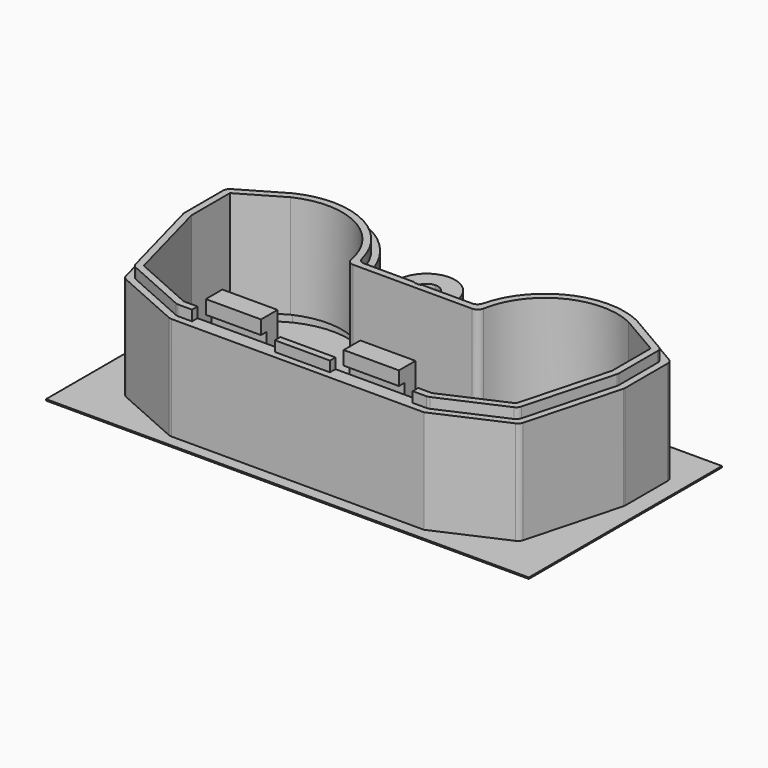
from build123d import *

# Parameters (mm, degrees)
F1_DEPTH       = 1.5
F2_DEPTH       = 15
F3_R           = 1
F5_DEPTH       = 1.5
F6_W           = 11
F6_H           = 1.5
F7_DEPTH       = 1
F8_W           = 10
F8_H           = 3
F9_DEPTH       = 1
F10_W          = 8
F10_H          = 1
F10_H_2        = 2
F11_DEPTH      = 5
F11_DEPTH_BACK = 2
F12_W          = 12
F12_H          = 1.5
F13_DEPTH      = 1
F14_W          = 70
F14_H          = 35
F15_DEPTH      = 0.2
F14_W_2        = 47
F14_H_2        = 15


with BuildPart() as f1:
    # F0 (on Top) → F1 (new body)
    with BuildSketch(Plane.XY):
        with BuildLine():
            ThreePointArc((0, 19.85), (-0.351781182, 19.8879361055), (-0.6873863542, 20))
            Line((-0.6873863542, 20), (-8.6247335107, 20))
            ThreePointArc((-8.6247335107, 20), (-14.7071371013, 28.2669276783), (-24.9698908295, 28.3836006819))
            Line((-24.9698908295, 28.3836006819), (-31.5, 24.5743703325))
            Line((-31.5, 24.5743703325), (-31.5, 16.8677394235))
            Line((-31.5, 16.8677394235), (-27.8417010277, 3.2797718121))
            Line((-27.8417010277, 3.2797718121), (-18.2122144504, -1))
            Line((-18.2122144504, -1), (0, -1))
            Line((0, -1), (18.2122144504, -1))
            Line((18.2122144504, -1), (27.8417010277, 3.2797718121))
            Line((27.8417010277, 3.2797718121), (31.5, 16.8677394235))
            Line((31.5, 16.8677394235), (31.5, 24.5743703325))
            Line((31.5, 24.5743703325), (24.9698908295, 28.3836006819))
            ThreePointArc((24.9698908295, 28.3836006819), (14.7071371013, 28.2669276783), (8.6247335107, 20))
            Line((8.6247335107, 20), (0.6873863542, 20))
            ThreePointArc((0.6873863542, 20), (0.351781182, 19.8879361055), (0, 19.85))
        make_face()
        with BuildLine():
            Line((0, 0), (-18, 0))
            Line((-18, 0), (-27, 4))
            Line((-27, 4), (-30.5, 17))
            Line((-30.5, 17), (-30.5, 24))
            Line((-30.5, 24), (-24.5, 27.5))
            ThreePointArc((-24.5, 27.5), (-14.7788745368, 27.1696331703), (-9.5, 19))
            Line((-9.5, 19), (0, 19))
            Line((0, 19), (9.5, 19))
            ThreePointArc((9.5, 19), (14.7788745368, 27.1696331703), (24.5, 27.5))
            Line((24.5, 27.5), (30.5, 24))
            Line((30.5, 24), (30.5, 17))
            Line((30.5, 17), (27, 4))
            Line((27, 4), (18, 0))
            Line((18, 0), (0, 0))
        make_face(mode=Mode.SUBTRACT)
    extrude(amount=F1_DEPTH)

    # F0 (on Top) + F1_face (on face) → F2 (join)
    with BuildSketch(Plane.XY):
        with BuildLine():
            Line((-28.6834020554, 2.5595436242), (-18.4244289009, -2))
            Line((-18.4244289009, -2), (0, -2))
            Line((0, -2), (18.4244289009, -2))
            Line((18.4244289009, -2), (28.6834020554, 2.5595436242))
            Line((28.6834020554, 2.5595436242), (32.5, 16.735478847))
            Line((32.5, 16.735478847), (32.5, 25.1487406649))
            Line((32.5, 25.1487406649), (25.4412317406, 29.2663554829))
            ThreePointArc((25.4412317406, 29.2663554829), (14.6485898576, 29.3519368457), (7.8123925294, 21))
            Line((7.8123925294, 21), (4.119769411, 21))
            ThreePointArc((4.119769411, 21), (3.1062437123, 24.2520446944), (0, 25.65))
            ThreePointArc((0, 25.65), (-3.1062437123, 24.2520446944), (-4.119769411, 21))
            Line((-4.119769411, 21), (-7.8123925294, 21))
            ThreePointArc((-7.8123925294, 21), (-14.6485898576, 29.3519368457), (-25.4412317406, 29.2663554829))
            Line((-25.4412317406, 29.2663554829), (-32.5, 25.1487406649))
            Line((-32.5, 25.1487406649), (-32.5, 16.735478847))
            Line((-32.5, 16.735478847), (-28.6834020554, 2.5595436242))
        make_face()
        with BuildLine():
            ThreePointArc((-0.6873863542, 20), (-1.6120638945, 21.851781182), (0, 23.15))
            ThreePointArc((0, 23.15), (1.6120638945, 21.851781182), (0.6873863542, 20))
            Line((0.6873863542, 20), (8.6247335107, 20))
            ThreePointArc((8.6247335107, 20), (14.7071371013, 28.2669276783), (24.9698908295, 28.3836006819))
            Line((24.9698908295, 28.3836006819), (31.5, 24.5743703325))
            Line((31.5, 24.5743703325), (31.5, 16.8677394235))
            Line((31.5, 16.8677394235), (27.8417010277, 3.2797718121))
            Line((27.8417010277, 3.2797718121), (18.2122144504, -1))
            Line((18.2122144504, -1), (0, -1))
            Line((0, -1), (-18.2122144504, -1))
            Line((-18.2122144504, -1), (-27.8417010277, 3.2797718121))
            Line((-27.8417010277, 3.2797718121), (-31.5, 16.8677394235))
            Line((-31.5, 16.8677394235), (-31.5, 24.5743703325))
            Line((-31.5, 24.5743703325), (-24.9698908295, 28.3836006819))
            ThreePointArc((-24.9698908295, 28.3836006819), (-14.7071371013, 28.2669276783), (-8.6247335107, 20))
            Line((-8.6247335107, 20), (-0.6873863542, 20))
        make_face(mode=Mode.SUBTRACT)
    with BuildSketch(Plane(origin=(0, 14.0196943872, 0), x_dir=(1, 0, 0), z_dir=(0, 0, -1))):
        with BuildLine():
            Line((31.5, -10.5546759452), (31.5, -2.8480450363))
            Line((31.5, -2.8480450363), (27.8417010277, 10.7399225751))
            Line((27.8417010277, 10.7399225751), (18.2122144504, 15.0196943872))
            Line((18.2122144504, 15.0196943872), (-18.2122144504, 15.0196943872))
            Line((-18.2122144504, 15.0196943872), (-27.8417010277, 10.7399225751))
            Line((-27.8417010277, 10.7399225751), (-31.5, -2.8480450363))
            Line((-31.5, -2.8480450363), (-31.5, -10.5546759452))
            Line((-31.5, -10.5546759452), (-24.9698908295, -14.3639062947))
            ThreePointArc((-24.9698908295, -14.3639062947), (-14.7071371013, -14.2472332911), (-8.6247335107, -5.9803056128))
            Line((-8.6247335107, -5.9803056128), (-0.6873863542, -5.9803056128))
            ThreePointArc((-0.6873863542, -5.9803056128), (0, -5.8303056128), (0.6873863542, -5.9803056128))
            Line((0.6873863542, -5.9803056128), (8.6247335107, -5.9803056128))
            ThreePointArc((8.6247335107, -5.9803056128), (14.7071371013, -14.2472332911), (24.9698908295, -14.3639062947))
            Line((24.9698908295, -14.3639062947), (31.5, -10.5546759452))
        make_face()
        with BuildLine():
            Line((-27, 10.0196943872), (-18, 14.0196943872))
            Line((-18, 14.0196943872), (18, 14.0196943872))
            Line((18, 14.0196943872), (27, 10.0196943872))
            Line((27, 10.0196943872), (30.5, -2.9803056128))
            Line((30.5, -2.9803056128), (30.5, -9.9803056128))
            Line((30.5, -9.9803056128), (24.5, -13.4803056128))
            ThreePointArc((24.5, -13.4803056128), (14.7788745368, -13.1499387831), (9.5, -4.9803056128))
            Line((9.5, -4.9803056128), (-9.5, -4.9803056128))
            ThreePointArc((-9.5, -4.9803056128), (-14.7788745368, -13.1499387831), (-24.5, -13.4803056128))
            Line((-24.5, -13.4803056128), (-30.5, -9.9803056128))
            Line((-30.5, -9.9803056128), (-30.5, -2.9803056128))
            Line((-30.5, -2.9803056128), (-27, 10.0196943872))
        make_face(mode=Mode.SUBTRACT)
    extrude(amount=-F2_DEPTH, dir=(0, 0, 1))

    # F3
    f3_edges = [f1.edges().sort_by_distance(p)[0] for p in [
        (7.812393, 21, -7.5),
        (-7.812393, 21, -7.5),
        (-4.119769, 21, -7.5),
        (4.119769, 21, -7.5),
        (32.5, 25.148741, -7.5),
        (32.5, 16.735479, -7.5),
        (28.683402, 2.559544, -7.5),
        (-18.424429, -2, -7.5),
        (-28.683402, 2.559544, -7.5),
        (-32.5, 16.735479, -7.5),
        (-32.5, 25.148741, -7.5),
        (31.5, 24.57437, 0.75),
        (31.5, 16.867739, 0.75),
        (27.841701, 3.279772, 0.75),
        (18.212214, -1, 0.75),
        (-18.212214, -1, 0.75),
        (-27.841701, 3.279772, 0.75),
        (-31.5, 16.867739, 0.75),
        (-31.5, 24.57437, 0.75),
        (-8.624734, 20, 0.75),
        (8.624734, 20, 0.75),
        (9.5, 19, 0.75),
        (9.5, 19, -7.5),
        (-9.5, 19, 0.75),
        (-9.5, 19, -7.5),
    ]]
    fillet(f3_edges, radius=F3_R)

    # F4 (on face) → F5 (cut)
    with BuildSketch(Plane(origin=(0, 0, -15), x_dir=(1, 0, 0), z_dir=(0, 0, -1))):
        with BuildLine():
            Line((27.8417010277, -3.2797718121), (18.2122144504, 1))
            Line((18.2122144504, 1), (-18.2122144504, 1))
            Line((-18.2122144504, 1), (-27.8417010277, -3.2797718121))
            Line((-27.8417010277, -3.2797718121), (-31.5, -16.8677394235))
            Line((-31.5, -16.8677394235), (-31.5, -24.5743703325))
            Line((-31.5, -24.5743703325), (-24.9698908295, -28.3836006819))
            ThreePointArc((-24.9698908295, -28.3836006819), (-14.7071371013, -28.2669276783), (-8.6247335107, -20))
            Line((-8.6247335107, -20), (8.6247335107, -20))
            ThreePointArc((8.6247335107, -20), (14.7071371013, -28.2669276783), (24.9698908295, -28.3836006819))
            Line((24.9698908295, -28.3836006819), (31.5, -24.5743703325))
            Line((31.5, -24.5743703325), (31.5, -16.8677394235))
            Line((31.5, -16.8677394235), (27.8417010277, -3.2797718121))
        make_face()
    extrude(amount=-F5_DEPTH, mode=Mode.SUBTRACT)

    # F6 (on face) → F7 (join, through all)
    with BuildSketch(Plane(origin=(0, 0, 0), x_dir=(-1, 0, 0), z_dir=(0, 1, 0))):
        with Locations((10, -14.25)):
            Rectangle(F6_W, F6_H)
        with Locations((-10, -14.25)):
            Rectangle(F6_W, F6_H)
    extrude(amount=-F7_DEPTH)

    # F8 (on face) → F9 (cut)
    with BuildSketch(Plane(origin=(0, 0, 0), x_dir=(-1, 0, 0), z_dir=(0, 1, 0))):
        with Locations((-10, -12.5)):
            Rectangle(F8_W, F8_H)
        with Locations((10, -12.5)):
            Rectangle(F8_W, F8_H)
    extrude(amount=-F9_DEPTH, mode=Mode.SUBTRACT)

    # F10 (on face) → F11 (join, two sides)
    with BuildSketch(Plane.XY.offset(1.5)) as f11_sk:
        with Locations((10, -0.5)):
            Rectangle(F10_W, F10_H)
        with Locations((-10, -0.5)):
            Rectangle(F10_W, F10_H)
        with Locations((-10, 1)):
            Rectangle(F10_W, F10_H_2)
        with Locations((10, 1)):
            Rectangle(F10_W, F10_H_2)
    extrude(amount=-F11_DEPTH)
    extrude(f11_sk.sketch, amount=F11_DEPTH_BACK)

    # F12 (on face) → F13 (cut)
    with BuildSketch(Plane.XZ.offset(1)):
        with Locations((-10, 0.75)):
            Rectangle(F12_W, F12_H)
        with Locations((10, 0.75)):
            Rectangle(F12_W, F12_H)
    extrude(amount=-F13_DEPTH, mode=Mode.SUBTRACT)


with BuildPart() as f15:
    # F14 (on face) → F15 (new body)
    with BuildSketch(Plane(origin=(0, 0, -15), x_dir=(1, 0, 0), z_dir=(0, 0, -1))):
        with Locations((0, -13.7961478531)):
            Rectangle(F14_W, F14_H)
        with BuildLine():
            Line((-28.2478394938, -2.3659602635), (-18.6183529165, 1.9138115486))
            ThreePointArc((-18.6183529165, 1.9138115486), (-18.419805938, 1.9782156073), (-18.2122144504, 2))
            Line((-18.2122144504, 2), (18.4244289009, 2))
            Line((18.4244289009, 2), (28.2478394938, -2.3659602635))
            ThreePointArc((28.2478394938, -2.3659602635), (28.6015059173, -2.629620653), (28.8073167862, -3.0197983387))
            Line((28.8073167862, -3.0197983387), (32.4656157585, -16.60776595))
            ThreePointArc((32.4656157585, -16.60776595), (32.4913666725, -16.7366206958), (32.5, -16.8677394235))
            Line((32.5, -16.8677394235), (32.5, -24.5743703325))
            ThreePointArc((32.5, -24.5743703325), (32.3671421526, -25.0724310589), (32.0038710255, -25.4381492334))
            Line((32.0038710255, -25.4381492334), (25.4412317406, -29.2663554829))
            ThreePointArc((25.4412317406, -29.2663554829), (14.9825022619, -29.5025835286), (8.0069708388, -21.7062518681))
            ThreePointArc((8.0069708388, -21.7062518681), (7.6453319845, -21.1957151836), (7.0510879824, -21))
            Line((7.0510879824, -21), (5.1256706878, -21))
            ThreePointArc((5.1256706878, -21), (4.4537657015, -21.2593626466), (4.1303948261, -21.9029126214))
            ThreePointArc((4.1303948261, -21.9029126214), (0, -25.65), (-4.1303948261, -21.9029126214))
            ThreePointArc((-4.1303948261, -21.9029126214), (-4.4537657015, -21.2593626466), (-5.1256706878, -21))
            Line((-5.1256706878, -21), (-7.0510879824, -21))
            ThreePointArc((-7.0510879824, -21), (-7.6453319845, -21.1957151836), (-8.0069708388, -21.7062518681))
            ThreePointArc((-8.0069708388, -21.7062518681), (-14.9825022619, -29.5025835286), (-25.4412317406, -29.2663554829))
            Line((-25.4412317406, -29.2663554829), (-32.0038710255, -25.4381492334))
            ThreePointArc((-32.0038710255, -25.4381492334), (-32.3671421526, -25.0724310589), (-32.5, -24.5743703325))
            Line((-32.5, -24.5743703325), (-32.5, -16.8677394235))
            ThreePointArc((-32.5, -16.8677394235), (-32.4913666725, -16.7366206958), (-32.4656157585, -16.60776595))
            Line((-32.4656157585, -16.60776595), (-28.8073167862, -3.0197983387))
            ThreePointArc((-28.8073167862, -3.0197983387), (-28.6015059173, -2.629620653), (-28.2478394938, -2.3659602635))
        make_face(mode=Mode.SUBTRACT)
    extrude(amount=F15_DEPTH)


with BuildPart() as f15b:
    # F14 (on face) → F15, piece 2 (new body)
    with BuildSketch(Plane(origin=(0, 0, -15), x_dir=(1, 0, 0), z_dir=(0, 0, -1))):
        with BuildLine():
            Line((-8.6247335107, -20), (-0.6873863542, -20))
            ThreePointArc((-0.6873863542, -20), (0, -23.15), (0.6873863542, -20))
            Line((0.6873863542, -20), (8.6247335107, -20))
            ThreePointArc((8.6247335107, -20), (14.7071371013, -28.2669276783), (24.9698908295, -28.3836006819))
            Line((24.9698908295, -28.3836006819), (31.5, -24.5743703325))
            Line((31.5, -24.5743703325), (31.5, -16.8677394235))
            Line((31.5, -16.8677394235), (27.8417010277, -3.2797718121))
            Line((27.8417010277, -3.2797718121), (18.2122144504, 1))
            Line((18.2122144504, 1), (15.5, 1))
            Line((15.5, 1), (15.5, 0))
            Line((15.5, 0), (4.5, 0))
            Line((4.5, 0), (4.5, 1))
            Line((4.5, 1), (-4.5, 1))
            Line((-4.5, 1), (-4.5, 0))
            Line((-4.5, 0), (-15.5, 0))
            Line((-15.5, 0), (-15.5, 1))
            Line((-15.5, 1), (-18.2122144504, 1))
            Line((-18.2122144504, 1), (-27.8417010277, -3.2797718121))
            Line((-27.8417010277, -3.2797718121), (-31.5, -16.8677394235))
            Line((-31.5, -16.8677394235), (-31.5, -24.5743703325))
            Line((-31.5, -24.5743703325), (-24.9698908295, -28.3836006819))
            ThreePointArc((-24.9698908295, -28.3836006819), (-14.7071371013, -28.2669276783), (-8.6247335107, -20))
        make_face()
        with Locations((-0.5, -10.4625395685)):
            Rectangle(F14_W_2, F14_H_2, mode=Mode.SUBTRACT)
    extrude(amount=F15_DEPTH)


solid = Compound([f1.part, f15.part, f15b.part])
